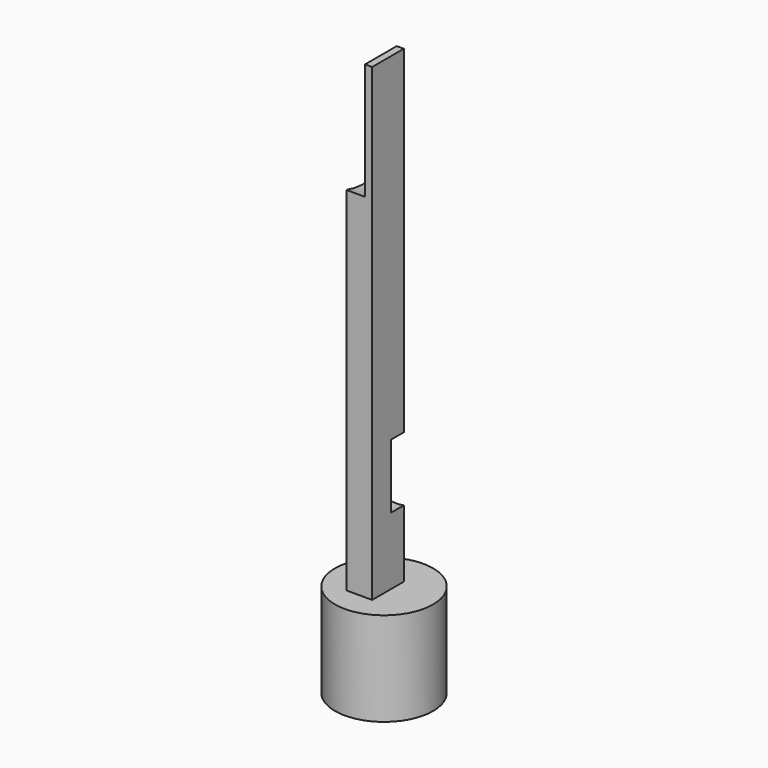
from build123d import *

# Parameters (mm, degrees)
F0_R      = 66.359491572
F1_DEPTH  = 101.6
F2_DEPTH  = 25.4
F3_W      = 9.6355099231
F3_H      = 53.5687487572
F4_DEPTH  = 635
F5_DEPTH  = 25.4
F9_DEPTH  = 25.4
F10_R     = 44.5685010644
F11_DEPTH = 25.4


# Not quite as in the source:
# - the program builds the solid bodies; features that only make, move or delete a surface that nothing else refers to are left out


with BuildPart() as f1:
    # F0 (on Top) → F1 (new body)
    with BuildSketch(Plane.XY):
        Circle(F0_R)
    extrude(amount=F1_DEPTH)

    # F2 (add): a face of the model
    f2_faces = [f1.faces().sort_by_distance(p)[0] for p in [
        (0, 0, 101.6),
    ]]
    extrude(f2_faces, amount=F2_DEPTH)

    # F3 (on face) → F4 (join)
    with BuildSketch(Plane.XY.offset(127)):
        with Locations((4.8177549616, -5.3717447445)):
            Rectangle(F3_W, F3_H)
    extrude(amount=F4_DEPTH)

    # F5 (add): a face of the model
    f5_faces = [f1.faces().sort_by_distance(p)[0] for p in [
        (0, -5.3717447445, 444.5),
    ]]
    extrude(f5_faces, amount=F5_DEPTH)

    # F8 (on face) → F9 (cut)
    with BuildSketch(Plane(origin=(-25.4, 0, 0), x_dir=(0, -1, 0), z_dir=(-1, 0, 0))):
        with BuildLine():
            Line((-21.4126296341, 762), (-21.4126296341, 601.4327447423))
            ThreePointArc((-21.4126296341, 601.4327447423), (5.5404234134, 599.4593595949), (32.1561191231, 604.1461558799))
            Line((32.1561191231, 604.1461558799), (32.1561191231, 762))
            Line((32.1561191231, 762), (-21.4126296341, 762))
        make_face()
        with BuildLine():
            ThreePointArc((32.1561191231, 604.1461558799), (88.0808871948, 643.7512740199), (109.5204650209, 708.8395953178))
            ThreePointArc((109.5204650209, 708.8395953178), (-69.4608202642, 793.5150150489), (-21.4126296341, 601.4327447423))
            Line((-21.4126296341, 601.4327447423), (-21.4126296341, 762))
            Line((-21.4126296341, 762), (32.1561191231, 762))
            Line((32.1561191231, 762), (32.1561191231, 604.1461558799))
        make_face()
    extrude(amount=-F9_DEPTH, mode=Mode.SUBTRACT)

    # F10 (on Front) → F11 (cut)
    with BuildSketch(Plane.XZ):
        with Locations((0, 261.4895105362)):
            Circle(F10_R)
    extrude(amount=-F11_DEPTH, mode=Mode.SUBTRACT)


solid = f1.part
